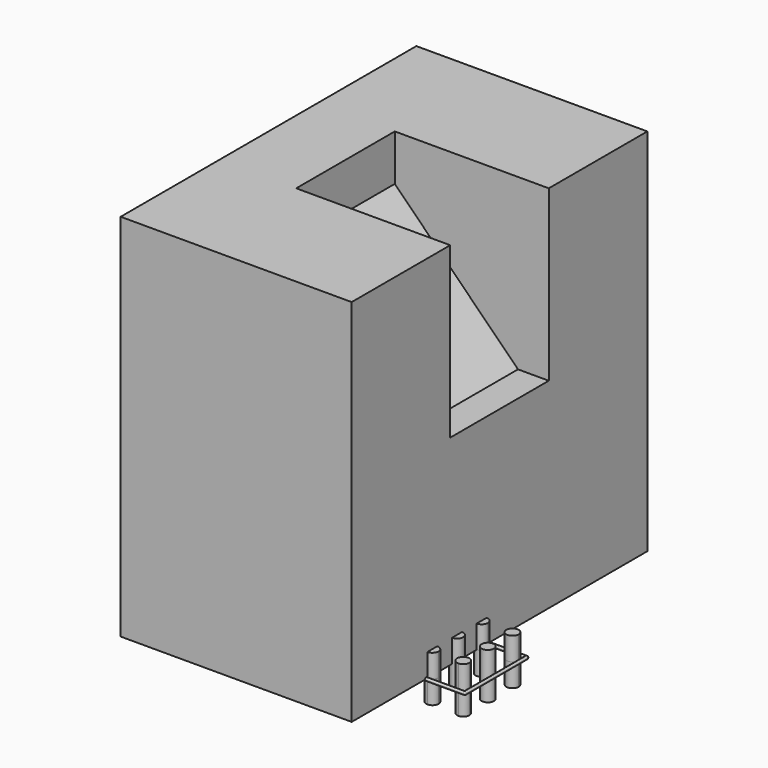
from build123d import *

# Parameters (mm, degrees)
F0_W     = 750
F0_H     = 1200
F1_DEPTH = 600
F3_DEPTH = 200
F4_R     = 100
F5_DEPTH = 919.2398155425
F7_DEPTH = 75
F6_R     = 20
F6_W     = 160
F6_H     = 260
F8_DEPTH = 5
F9_R     = 4.99999


# Not quite as in the source:
# - a fillet or chamfer is up to 0.001 mm smaller than in the source, because OpenCascade refuses the exact size


with BuildPart() as f1:
    # F0 (on Front) → F1 (new body, symmetric)
    with BuildSketch(Plane.XZ):
        with Locations((-375, 600)):
            Rectangle(F0_W, F0_H)
    extrude(amount=F1_DEPTH, both=True)

    # F2 (on Front) → F3 (cut, symmetric)
    with BuildSketch(Plane.XZ):
        Polygon((0, 650), (0, 1200), (-500, 1200), (-500, 1050), (-100, 650), align=None)
    extrude(amount=F3_DEPTH, both=True, mode=Mode.SUBTRACT)

    # F4 (on face) → F5 (cut, through all)
    with BuildSketch(Plane(origin=(275, 0, 275), x_dir=(0.7071067812, 0, -0.7071067812), z_dir=(0.7071067812, 0, 0.7071067812))):
        with Locations((-813.1728008391, 0)):
            Circle(F4_R)
    extrude(amount=-F5_DEPTH, mode=Mode.SUBTRACT)


with BuildPart() as f7:
    # F6 (on Top) → F7 (new body, symmetric)
    with BuildSketch(Plane.XY):
        with BuildLine():
            ThreePointArc((20.2996149659, -172.657354176), (0.2996149659, -152.657354176), (-19.7003850341, -172.657354176))
            ThreePointArc((-19.7003850341, -172.657354176), (0.2996149659, -192.657354176), (20.2996149659, -172.657354176))
        make_face()
    extrude(amount=F7_DEPTH, both=True)


with BuildPart() as f7b:
    # F6 (on Top) → F7, piece 2 (new body, symmetric)
    with BuildSketch(Plane.XY):
        with Locations((100.2996149659, -172.657354176)):
            Circle(F6_R)
    extrude(amount=F7_DEPTH, both=True)


with BuildPart() as f7c:
    # F6 (on Top) → F7, piece 3 (new body, symmetric)
    with BuildSketch(Plane.XY):
        with BuildLine():
            ThreePointArc((120.2996149659, -72.657354176), (114.4417505896, -58.5152185523), (100.2996149659, -52.657354176))
            ThreePointArc((100.2996149659, -52.657354176), (86.1574793422, -86.7994897998), (120.2996149659, -72.657354176))
        make_face()
    extrude(amount=F7_DEPTH, both=True)


with BuildPart() as f7d:
    # F6 (on Top) → F7, piece 4 (new body, symmetric)
    with BuildSketch(Plane.XY):
        with BuildLine():
            ThreePointArc((20.2996149659, -72.657354176), (14.4417505732, -58.5152185358), (0.2996149193, -52.657354176))
            ThreePointArc((0.2996149193, -52.657354176), (-13.8425206743, -58.5152185688), (-19.7003850341, -72.657354176))
            ThreePointArc((-19.7003850341, -72.657354176), (0.2996149659, -92.657354176), (20.2996149659, -72.657354176))
        make_face()
    extrude(amount=F7_DEPTH, both=True)


with BuildPart() as f7e:
    # F6 (on Top) → F7, piece 5 (new body, symmetric)
    with BuildSketch(Plane.XY):
        with BuildLine():
            ThreePointArc((20.2996149659, -272.657354176), (0.2996149659, -252.657354176), (-19.7003850341, -272.657354176))
            ThreePointArc((-19.7003850341, -272.657354176), (-13.8425206578, -286.7994897998), (0.2996149659, -292.657354176))
            ThreePointArc((0.2996149659, -292.657354176), (14.4417505896, -286.7994897998), (20.2996149659, -272.657354176))
        make_face()
    extrude(amount=F7_DEPTH, both=True)


with BuildPart() as f7f:
    # F6 (on Top) → F7, piece 6 (new body, symmetric)
    with BuildSketch(Plane.XY):
        with BuildLine():
            ThreePointArc((100.2996149659, -292.657354176), (114.4417505896, -286.7994897998), (120.2996149659, -272.657354176))
            ThreePointArc((120.2996149659, -272.657354176), (86.1574793422, -258.5152185523), (100.2996149659, -292.657354176))
        make_face()
    extrude(amount=F7_DEPTH, both=True)


with BuildPart() as f8:
    # F6 (on Top) → F8 (new body, symmetric)
    with BuildSketch(Plane.XY):
        with Locations((50.2996149659, -172.657354176)):
            Rectangle(F6_W, F6_H)
        Polygon((-19.7003850341, -72.657354176), (-19.7003850341, -52.657354176), (0.2996149193, -52.657354176), (100.2996149659, -52.657354176), (120.2996149659, -52.657354176), (120.2996149659, -72.657354176), (120.2996149659, -172.657354176), (120.2996149659, -272.657354176), (120.2996149659, -292.657354176), (100.2996149659, -292.657354176), (0.2996149659, -292.657354176), (-19.7003850341, -292.657354176), (-19.7003850341, -272.657354176), (-19.7003850341, -172.657354176), align=None, mode=Mode.SUBTRACT)
    extrude(amount=F8_DEPTH, both=True)

    # F9 (radius 5 in the source; OpenCascade refuses exactly that, so slightly less here)
    f9_edges = [f8.edges().sort_by_distance(p)[0] for p in [
        (-29.700385, -172.657354, 5),
        (-19.700385, -172.657354, 5),
        (-29.700385, -172.657354, -5),
        (50.299615, -302.657354, -5),
        (50.299615, -302.657354, 5),
        (50.299615, -292.657354, 5),
        (50.299615, -292.657354, -5),
        (-19.700385, -172.657354, -5),
        (120.299615, -172.657354, -5),
        (130.299615, -172.657354, -5),
        (130.299615, -172.657354, 5),
        (120.299615, -172.657354, 5),
        (130.299615, -302.657354, 0),
        (-29.700385, -302.657354, 0),
        (50.299615, -42.657354, 5),
        (50.299615, -42.657354, -5),
        (130.299615, -42.657354, 0),
        (50.299615, -52.657354, 5),
        (-29.700385, -42.657354, 0),
        (50.299615, -52.657354, -5),
    ]]
    fillet(f9_edges, radius=F9_R)


solid = Compound([f1.part, f7.part, f7b.part, f7c.part, f7d.part, f7e.part, f7f.part, f8.part])
